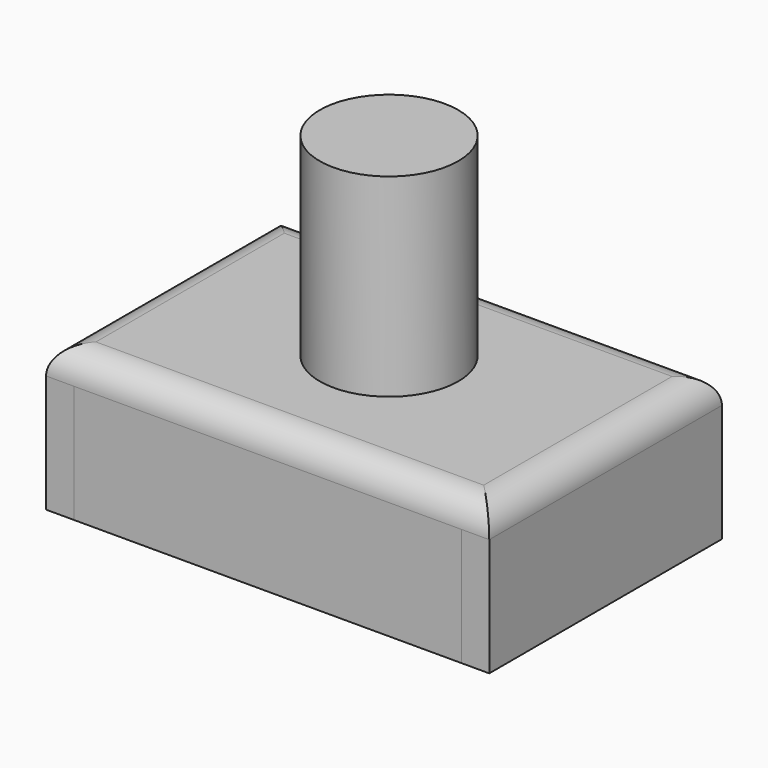
from build123d import *

# Parameters (mm, degrees)
F0_W      = 18
F0_H      = 17
F0_W_2    = 14
F0_H_2    = 13
F1_DEPTH  = 8
F2_W      = 9
F2_H      = 13
F3_DEPTH  = 2
F5_W      = 13
F5_H      = 12
F6_DEPTH  = 6
F7_R      = 3.5
F8_DEPTH  = 5
F9_R      = 3
F10_DEPTH = 10
F11_W     = 5
F11_H     = 17
F11_R     = 1.15
F12_DEPTH = 2
F13_W     = 5
F13_H     = 4
F14_DEPTH = 6
F15_W     = 28
F15_H     = 8.5
F16_DEPTH = 2
F17_W     = 21
F17_H     = 8.5
F18_DEPTH = 2
F19_W     = 28
F19_H     = 8.5
F20_DEPTH = 2
F21_W     = 21
F21_H     = 8.5
F22_DEPTH = 2
F23_R     = 1.15
F24_DEPTH = 5
F25_W     = 32
F25_H     = 21
F26_DEPTH = 2
F27_R     = 3.75
F28_DEPTH = 5
F29_R     = 5
F30_DEPTH = 14
F31_R     = 1.99999


# Not quite as in the source:
# - a fillet or chamfer is up to 0.001 mm smaller than in the source, because OpenCascade refuses the exact size


with BuildPart() as f1:
    # F0 (on Top) → F1 (new body)
    with BuildSketch(Plane.XY):
        with Locations((7, -6.5)):
            Rectangle(F0_W, F0_H)
        with Locations((7, -6.5)):
            Rectangle(F0_W_2, F0_H_2, mode=Mode.SUBTRACT)
    extrude(amount=F1_DEPTH)

    # F2 (on face) → F3 (join)
    with BuildSketch(Plane(origin=(0, 0, 0), x_dir=(1, 0, 0), z_dir=(0, 0, -1))):
        with Locations((7, 6.5)):
            Rectangle(F2_W, F2_H)
    extrude(amount=-F3_DEPTH)

    # F11 (on Top) → F12 (join)
    with BuildSketch(Plane.XY):
        with Locations((-4.5, -6.5)):
            Rectangle(F11_W, F11_H)
        with Locations((-4.35, -11.85)):
            Circle(F11_R, mode=Mode.SUBTRACT)
        with Locations((-4.35, -1.15)):
            Circle(F11_R, mode=Mode.SUBTRACT)
        with Locations((18.5, -6.5)):
            Rectangle(F11_W, F11_H)
        with Locations((18.35, -11.85)):
            Circle(F11_R, mode=Mode.SUBTRACT)
        with Locations((18.35, -1.15)):
            Circle(F11_R, mode=Mode.SUBTRACT)
    extrude(amount=F12_DEPTH)

    # F13 (on face) → F14 (join)
    with BuildSketch(Plane.XY.offset(2)):
        with Locations((-4.5, -6.5)):
            Rectangle(F13_W, F13_H)
        with Locations((18.5, -6.5)):
            Rectangle(F13_W, F13_H)
    extrude(amount=F14_DEPTH)


with BuildPart() as f6:
    # F5 (on face) → F6 (new body)
    with BuildSketch(Plane.XY.offset(2)):
        with Locations((6.9626439363, -6.4136818983)):
            Rectangle(F5_W, F5_H)
    extrude(amount=F6_DEPTH)


with BuildPart() as f8:
    # F7 (on face) → F8 (new body)
    with BuildSketch(Plane.XY.offset(8)):
        with Locations((6.9626439363, -6)):
            Circle(F7_R)
    extrude(amount=F8_DEPTH)


with BuildPart() as f10:
    # F9 (on face) → F10 (new body)
    with BuildSketch(Plane.XY.offset(13)):
        with Locations((6.9626439363, -6)):
            Circle(F9_R)
    extrude(amount=F10_DEPTH)


with BuildPart() as f16:
    # F15 (on face) → F16 (new body)
    with BuildSketch(Plane.XZ.offset(15)):
        with Locations((7, 4.25)):
            Rectangle(F15_W, F15_H)
    extrude(amount=F16_DEPTH)


with BuildPart() as f18:
    # F17 (on face) → F18 (new body)
    with BuildSketch(Plane.YZ.offset(21)):
        with Locations((-6.5, 4.25)):
            Rectangle(F17_W, F17_H)
    extrude(amount=F18_DEPTH)


with BuildPart() as f20:
    # F19 (on face) → F20 (new body)
    with BuildSketch(Plane(origin=(0, 2, 0), x_dir=(-1, 0, 0), z_dir=(0, 1, 0))):
        with Locations((-7, 4.25)):
            Rectangle(F19_W, F19_H)
    extrude(amount=F20_DEPTH)


with BuildPart() as f22:
    # F21 (on face) → F22 (new body)
    with BuildSketch(Plane(origin=(-7, 0, 0), x_dir=(0, -1, 0), z_dir=(-1, 0, 0))):
        with Locations((6.5, 4.25)):
            Rectangle(F21_W, F21_H)
    extrude(amount=F22_DEPTH)


with BuildPart() as f24_tool:
    # F23 (on face) → F24 (new body)
    with BuildSketch(Plane(origin=(-9, 0, 0), x_dir=(0, -1, 0), z_dir=(-1, 0, 0))):
        with Locations((6.5, 4.85)):
            Circle(F23_R)
    extrude(amount=-F24_DEPTH)


with BuildPart() as f1_1:
    add(f1.part)

    # F24: cut by f24_tool
    add(f24_tool.part, mode=Mode.SUBTRACT)


with BuildPart() as f22_1:
    add(f22.part)

    # F24: cut by f24_tool
    add(f24_tool.part, mode=Mode.SUBTRACT)


with BuildPart() as f26:
    # F25 (on face) → F26 (new body)
    with BuildSketch(Plane.XY.offset(8.5)):
        with Locations((7, -6.5)):
            Rectangle(F25_W, F25_H)
    extrude(amount=F26_DEPTH)

    # F27 (on face) → F28 (cut)
    with BuildSketch(Plane.XY.offset(13)):
        with Locations((6.9626439363, -6)):
            Circle(F27_R)
    extrude(amount=-F28_DEPTH, mode=Mode.SUBTRACT)

    # F31 (radius 2 in the source; OpenCascade refuses exactly that, so slightly less here)
    f31_edges = [f26.edges().sort_by_distance(p)[0] for p in [
        (-9, -6.5, 10.5),
        (7, 4, 10.5),
        (7, -17, 10.5),
        (23, -6.5, 10.5),
    ]]
    fillet(f31_edges, radius=F31_R)


with BuildPart() as f30:
    # F29 (on face) → F30 (new body)
    with BuildSketch(Plane.XY.offset(10.5)):
        with Locations((6.9626439363, -6)):
            Circle(F29_R)
    extrude(amount=F30_DEPTH)


solid = Compound([f6.part, f8.part, f10.part, f16.part, f18.part, f20.part, f1_1.part, f22_1.part, f26.part, f30.part])
